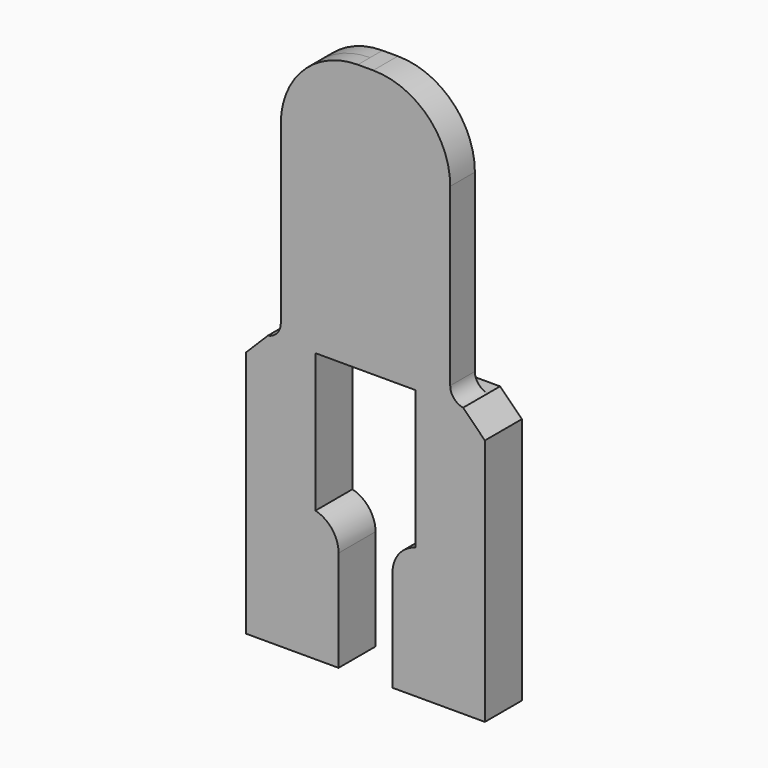
from build123d import *

# Parameters (mm, degrees)
F3_DEPTH    = 2
F4_W        = 1
F4_H        = 17.3801295459
F5_DEPTH    = 13.251
F6_R        = 5
F7_T1_DEPTH = 1
F8_T1_DEPTH = 11.6824583655
F9_DEPTH    = 1


# Not quite as in the source:
# - a fillet or chamfer that OpenCascade refuses, or shapes differently, is made with other operations: its cross-section is extruded or revolved along the edge and cut away or added


with BuildPart() as f3:
    # F2 (on line) → F3 (new body)
    with BuildSketch(Plane(origin=(0, -12, 0), x_dir=(-1, 0, 0), z_dir=(0, 1, 0))):
        Polygon((-7.75, 0), (-1.75, 0), (-1.75, 8.5), (-3.25, 8.5), (-3.25, 17.5), (-5.5, 17.5), (-6.3357864376, 17.5), (-7.75, 16.0857864376), align=None)
        Polygon((5.5, 17.5), (3.25, 17.5), (3.25, 8.5), (1.75, 8.5), (1.75, 0), (7.75, 0), (7.75, 16.0857864376), (6.3357864376, 17.5), align=None)
        Polygon((-5.5, 17.5), (-3.25, 17.5), (3.25, 17.5), (5.5, 17.5), (5.5, 34.8801295459), (0, 34.8801295459), (-5.5, 34.8801295459), align=None)
    extrude(amount=F3_DEPTH)

    # F4 (on face) → F5 (cut, through all)
    with BuildSketch(Plane.YZ.offset(5.5)):
        with Locations((-10.5, 26.190064773)):
            Rectangle(F4_W, F4_H)
    extrude(amount=-F5_DEPTH, mode=Mode.SUBTRACT)

    # F6
    f6_edges = [f3.edges().sort_by_distance(p)[0] for p in [
        (5.5, -11.5, 34.88013),
        (-5.5, -11.5, 34.88013),
    ]]
    fillet(f6_edges, radius=F6_R)

    # F7: fillet of radius 1 on 2 edges, made by hand

    # F7_s2 → F7_t1 (join)
    with BuildSketch(Plane.XZ.offset(11)):
        with BuildLine():
            ThreePointArc((5.5, 18.4864248101), (5.7370407736, 17.8399782007), (6.3357864376, 17.5))
            Line((6.3357864376, 17.5), (5.5, 17.5))
            Line((5.5, 17.5), (5.5, 18.4864248101))
        make_face()
        with BuildLine():
            ThreePointArc((-6.3357864376, 17.5), (-5.7370407736, 17.8399782007), (-5.5, 18.4864248101))
            Line((-5.5, 18.4864248101), (-5.5, 17.5))
            Line((-5.5, 17.5), (-6.3357864376, 17.5))
        make_face()
    extrude(amount=F7_T1_DEPTH)

    # F8: fillet of radius 2 on 2 edges, made by hand

    # F8_s2 → F8_t1 (cut)
    with BuildSketch(Plane.XZ.offset(5.1587708172)):
        with BuildLine():
            ThreePointArc((3.25, 8.5), (2.1688611699, 7.7882531983), (1.75, 6.5635083269))
            Line((1.75, 6.5635083269), (1.75, 8.5))
            Line((1.75, 8.5), (3.25, 8.5))
        make_face()
        with BuildLine():
            ThreePointArc((-1.75, 6.5635083269), (-2.1688611699, 7.7882531983), (-3.25, 8.5))
            Line((-3.25, 8.5), (-1.75, 8.5))
            Line((-1.75, 8.5), (-1.75, 6.5635083269))
        make_face()
    extrude(amount=F8_T1_DEPTH, mode=Mode.SUBTRACT)

    # F9 (add): a face of the model
    f9_faces = [f3.faces().sort_by_distance(p)[0] for p in [
        (-5.4458267789, -12, 17.5932359202),
    ]]
    extrude(f9_faces, amount=F9_DEPTH)


solid = f3.part
